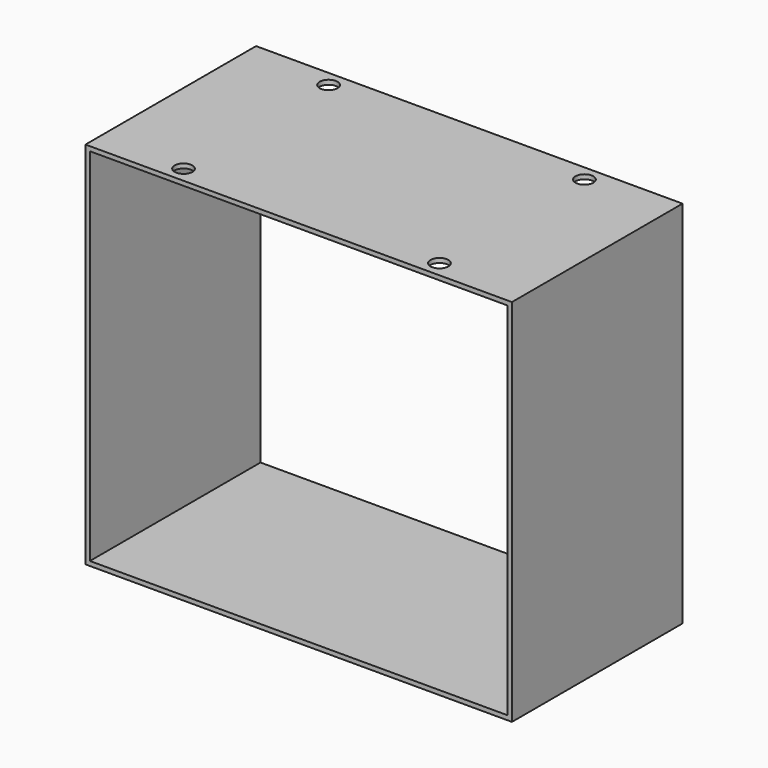
from build123d import *

# Parameters (mm, degrees)
F0_W     = 304.8
F0_H     = 152.4
F1_DEPTH = 3.175
F4_D     = 12.7
F5_W     = 3.175
F5_H     = 152.4
F6_DEPTH = 257.81
F7_W     = 304.8
F7_H     = 152.4
F8_DEPTH = 3.175


# Not quite as in the source:
# - a length typed as a fraction of an inch, garbled in the dataset ("3 / 203.2 mm" for 3/8 in), is restored


with BuildPart() as f1:
    # F0 (on Top) → F1 (new body)
    with BuildSketch(Plane.XY):
        Rectangle(F0_W, F0_H)
    extrude(amount=F1_DEPTH)

    # F4 (through all)
    with Locations(Plane.XY.offset(3.175)):
        with Locations((-91.44, 64.77), (-91.44, -64.77), (91.44, -64.77), (91.44, 64.77)):
            Hole(F4_D / 2)

    # F5 (on face) → F6 (join)
    with BuildSketch(Plane(origin=(0, 0, 0), x_dir=(1, 0, 0), z_dir=(0, 0, -1))):
        with Locations((-150.8125, 0)):
            Rectangle(F5_W, F5_H)
        with Locations((150.8125, 0)):
            Rectangle(F5_W, F5_H)
    extrude(amount=F6_DEPTH)

    # F7 (on face) → F8 (join)
    with BuildSketch(Plane(origin=(0, 0, -257.81), x_dir=(1, 0, 0), z_dir=(0, 0, -1))):
        Rectangle(F7_W, F7_H)
    extrude(amount=F8_DEPTH)


solid = f1.part
